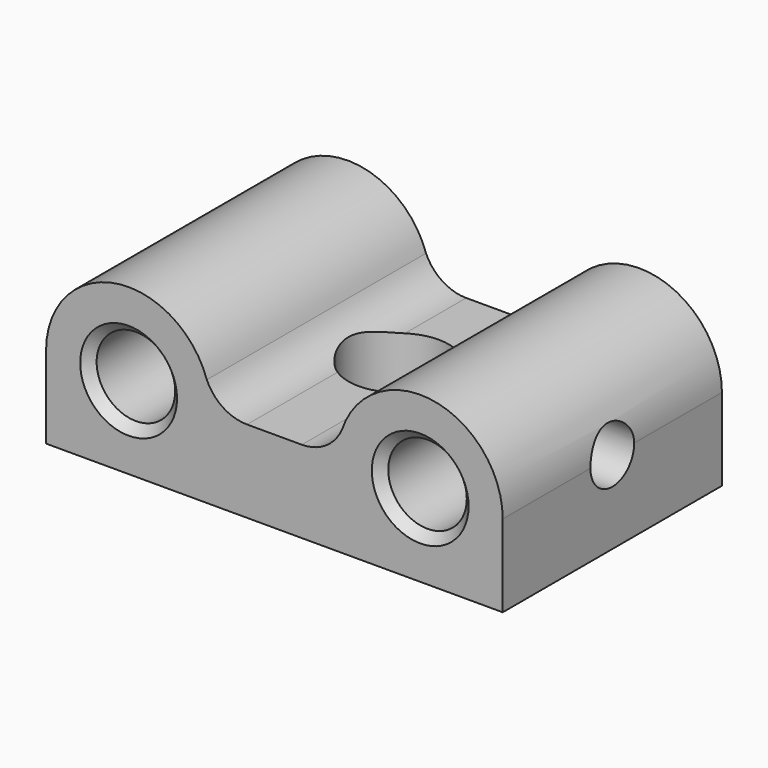
from build123d import *

# Parameters (mm, degrees)
F0_R     = 2.15
F1_DEPTH = 15
F3_D     = 5.5
F4_SIZE  = 0.5
F6_D     = 3
F6_DEPTH = 3
F6_TIP   = 0.9012909285
F8_D     = 3
F8_DEPTH = 3
F8_TIP   = 0.9012909285


with BuildPart() as f1:
    # F0 (on Front) → F1 (new body)
    with BuildSketch(Plane.XZ):
        with BuildLine():
            Line((-12.5, 4.5), (-12.5, 0))
            Line((-12.5, 0), (0, 0))
            Line((0, 0), (12.5, 0))
            Line((12.5, 0), (12.5, 4.5))
            ThreePointArc((12.5, 4.5), (8.7106121428, 8.9589284982), (3.6988942602, 5.9383014856))
            ThreePointArc((3.6988942602, 5.9383014856), (2.8137586471, 4.8915084722), (1.5, 4.5))
            Line((1.5, 4.5), (0, 4.5))
            Line((0, 4.5), (-1.5, 4.5))
            ThreePointArc((-1.5, 4.5), (-2.8137586471, 4.8915084722), (-3.6988942602, 5.9383014856))
            ThreePointArc((-3.6988942602, 5.9383014856), (-8.7106121428, 8.9589284982), (-12.5, 4.5))
        make_face()
        with Locations((-7.9819214904, 4.5)):
            Circle(F0_R, mode=Mode.SUBTRACT)
        with Locations((7.9819214904, 4.5)):
            Circle(F0_R, mode=Mode.SUBTRACT)
    extrude(amount=F1_DEPTH)

    # F3 (through all)
    with Locations(Plane(origin=(0, 0, 0), x_dir=(1, 0, 0), z_dir=(0, 0, -1))):
        with Locations((0, 6.5)):
            Hole(F3_D / 2)

    # F4
    f4_edges = [f1.edges().sort_by_distance(p)[0] for p in [
        (-10.131921, 0, 4.5),
        (5.831921, 0, 4.5),
        (-10.131921, -15, 4.5),
        (5.831921, -15, 4.5),
        (-2.75, -6.5, 0),
    ]]
    chamfer(f4_edges, length=F4_SIZE)

    # F6
    with Locations(Plane(origin=(-12.5, 0, 0), x_dir=(0, -1, 0), z_dir=(-1, 0, 0))):
        with Locations((7.5, 4.5)):
            Hole(F6_D / 2, depth=F6_DEPTH)
            with Locations((0, 0, -(F6_DEPTH + F6_TIP / 2))):  # 118° drill point
                Cone(0, F6_D / 2, F6_TIP, mode=Mode.SUBTRACT)

    # F8
    with Locations(Plane.YZ.offset(12.5)):
        with Locations((-7.5, 4.5)):
            Hole(F8_D / 2, depth=F8_DEPTH)
            with Locations((0, 0, -(F8_DEPTH + F8_TIP / 2))):  # 118° drill point
                Cone(0, F8_D / 2, F8_TIP, mode=Mode.SUBTRACT)


solid = f1.part
